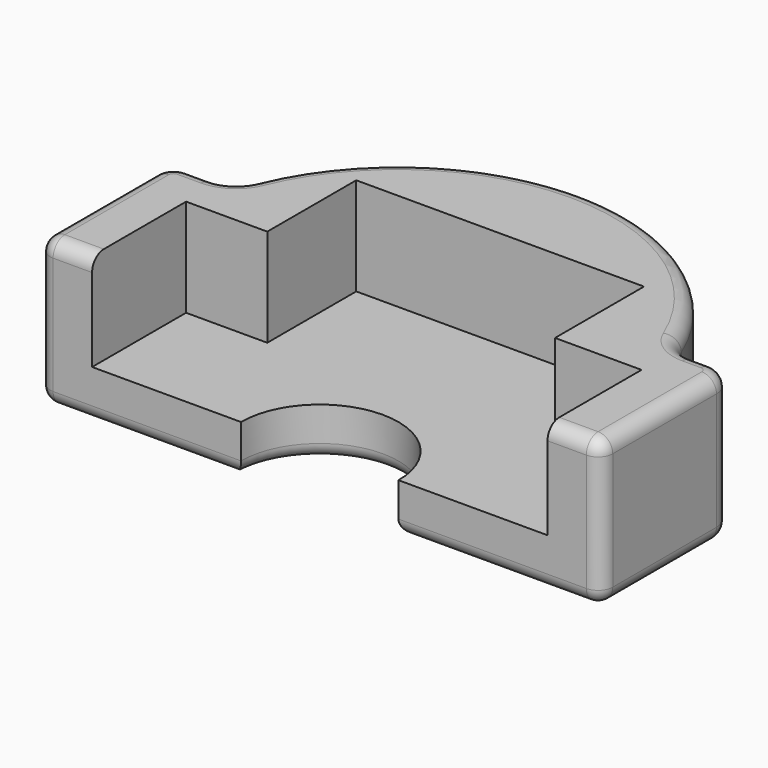
from build123d import *

# Parameters (mm, degrees)
F1_DEPTH     = 3.81
F2_R         = 0.762
F3_R         = 0.508
F4_R         = 0.381
F5_T1_DEPTH  = 0.6101247647
F5_T3_DEPTH  = 3.3655
F5_T5_DEPTH  = 5.8289214894
F5_T7_DEPTH  = 0.4831247647
F5_T9_DEPTH  = 5.8289214894
F5_T11_DEPTH = 3.048
F5_S15_W     = 0.381
F5_S15_H     = 0.381
F5_T16_DEPTH = 0.381
F5_S21_W     = 0.381
F5_S21_H     = 0.381
F5_T22_DEPTH = 0.381
F5_S27_W     = 0.381
F5_S27_H     = 0.381
F5_T28_DEPTH = 0.381
F5_S33_W     = 0.381
F5_S33_H     = 0.381
F5_T34_DEPTH = 0.381
F5_T38_ANGLE = 90
F5_T40_ANGLE = 67.60378922
F5_T42_ANGLE = 135.20757844
F5_T44_ANGLE = 67.60378922
F5_T46_ANGLE = 233.4571121673
F5_T48_ANGLE = 90
F7_DEPTH     = 2.54


# Not quite as in the source:
# - a fillet or chamfer that OpenCascade refuses, or shapes differently, is made with other operations: its cross-section is extruded or revolved along the edge and cut away or added


with BuildPart() as f1:
    # F0 (on Top) → F1 (new body)
    with BuildSketch(Plane.XY):
        with BuildLine():
            Line((0, -4.2545), (0, -8.509))
            Line((0, -8.509), (5.2574214894, -8.509))
            ThreePointArc((5.2574214894, -8.509), (7.3025, -6.4639214894), (9.3475785106, -8.509))
            Line((9.3475785106, -8.509), (14.605, -8.509))
            Line((14.605, -8.509), (14.605, -4.2545))
            Line((14.605, -4.2545), (13.081, -4.2545))
            ThreePointArc((13.081, -4.2545), (7.366, -0.0716128896), (1.651, -4.2545))
            Line((1.651, -4.2545), (0, -4.2545))
        make_face()
    extrude(amount=F1_DEPTH)

    # F2
    f2_edges = [f1.edges().sort_by_distance(p)[0] for p in [
        (13.081, -4.2545, 1.905),
        (1.651, -4.2545, 1.905),
    ]]
    fillet(f2_edges, radius=F2_R)

    # F3
    f3_edges = [f1.edges().sort_by_distance(p)[0] for p in [
        (0, -4.2545, 1.905),
        (14.605, -4.2545, 1.905),
    ]]
    fillet(f3_edges, radius=F3_R)

    # F4
    f4_edges = [f1.edges().sort_by_distance(p)[0] for p in [
        (0.813062, -4.2545, 0),
        (0.14879, -4.40329, 0),
        (1.542043, -4.125696, 0),
        (0, -6.63575, 0),
        (7.366, -0.071613, 0),
        (2.628711, -8.509, 0),
        (13.189957, -4.125696, 0),
        (7.3025, -6.463921, 0),
        (13.855438, -4.2545, 0),
        (11.976289, -8.509, 0),
        (14.45621, -4.40329, 0),
        (14.605, -6.63575, 0),
    ]]
    fillet(f4_edges, radius=F4_R)

    # F5: fillet of radius 0.381 on 14 edges, made by hand

    # F5_s2 → F5_t1 (cut)
    with BuildSketch(Plane.YZ.offset(0.508)):
        with BuildLine():
            ThreePointArc((-4.2545, 3.429), (-4.3660923164, 3.6984076836), (-4.6355, 3.81))
            Line((-4.6355, 3.81), (-4.2545, 3.81))
            Line((-4.2545, 3.81), (-4.2545, 3.429))
        make_face()
    extrude(amount=F5_T1_DEPTH, mode=Mode.SUBTRACT)

    # F5_s4 → F5_t3 (cut)
    with BuildSketch(Plane.XZ.offset(4.7625)):
        with BuildLine():
            ThreePointArc((0.381, 3.81), (0.1115923164, 3.6984076836), (0, 3.429))
            Line((0, 3.429), (0, 3.81))
            Line((0, 3.81), (0.381, 3.81))
        make_face()
        with BuildLine():
            ThreePointArc((14.224, 3.81), (14.4934076836, 3.6984076836), (14.605, 3.429))
            Line((14.605, 3.429), (14.605, 3.81))
            Line((14.605, 3.81), (14.224, 3.81))
        make_face()
    extrude(amount=F5_T3_DEPTH, mode=Mode.SUBTRACT)

    # F5_s6 → F5_t5 (cut)
    with BuildSketch(Plane.YZ.offset(0.381)):
        with BuildLine():
            ThreePointArc((-8.128, 3.81), (-8.3974076836, 3.6984076836), (-8.509, 3.429))
            Line((-8.509, 3.429), (-8.509, 3.81))
            Line((-8.509, 3.81), (-8.128, 3.81))
        make_face()
    extrude(amount=F5_T5_DEPTH, mode=Mode.SUBTRACT)

    # F5_s8 → F5_t7 (cut)
    with BuildSketch(Plane.YZ.offset(13.6138752353)):
        with BuildLine():
            ThreePointArc((-4.6355, 3.81), (-4.3660923164, 3.6984076836), (-4.2545, 3.429))
            Line((-4.2545, 3.429), (-4.2545, 3.81))
            Line((-4.2545, 3.81), (-4.6355, 3.81))
        make_face()
    extrude(amount=F5_T7_DEPTH, mode=Mode.SUBTRACT)

    # F5_s10 → F5_t9 (cut)
    with BuildSketch(Plane.YZ.offset(8.3950785106)):
        with BuildLine():
            ThreePointArc((-8.128, 3.81), (-8.3974076836, 3.6984076836), (-8.509, 3.429))
            Line((-8.509, 3.429), (-8.509, 3.81))
            Line((-8.509, 3.81), (-8.128, 3.81))
        make_face()
    extrude(amount=F5_T9_DEPTH, mode=Mode.SUBTRACT)

    # F5_s12 → F5_t11 (cut)
    with BuildSketch(Plane.XY.offset(0.381)):
        with BuildLine():
            ThreePointArc((0, -8.128), (0.1115923164, -8.3974076836), (0.381, -8.509))
            Line((0.381, -8.509), (0, -8.509))
            Line((0, -8.509), (0, -8.128))
        make_face()
        with BuildLine():
            ThreePointArc((14.224, -8.509), (14.4934076836, -8.3974076836), (14.605, -8.128))
            Line((14.605, -8.128), (14.605, -8.509))
            Line((14.605, -8.509), (14.224, -8.509))
        make_face()
    extrude(amount=F5_T11_DEPTH, mode=Mode.SUBTRACT)


with BuildPart() as f5_tool14:
    # F5_s15 → F5_t16 (new body)
    with BuildSketch(Plane.XZ.offset(8.128)):
        with Locations((14.4145, 0.1905)):
            Rectangle(F5_S15_W, F5_S15_H)
    extrude(amount=F5_T16_DEPTH)

    # F5_s17 → F5_t18 (revolve, cut)
    with BuildSketch(Plane(origin=(14.224, -8.128, 0.381), x_dir=(-0.7071067812, 0, 0.7071067812), z_dir=(0.7071067812, 0, 0.7071067812))):
        with BuildLine():
            ThreePointArc((0, -0.381), (0.381, 0), (0, 0.381))
            Line((0, 0.381), (0, -0.381))
        make_face()
    revolve(axis=Axis((14.224, -8.128, 0.381), (0, -1, 0)), mode=Mode.SUBTRACT)


with BuildPart() as f1_1:
    add(f1.part)

    # F5_t13: cut F5_tool14
    add(f5_tool14.part, mode=Mode.SUBTRACT)


with BuildPart() as f5_tool20:
    # F5_s21 → F5_t22 (new body)
    with BuildSketch(Plane.YZ.offset(0.381)):
        with Locations((-8.3185, 0.1905)):
            Rectangle(F5_S21_W, F5_S21_H)
    extrude(amount=-F5_T22_DEPTH)

    # F5_s23 → F5_t24 (revolve, cut)
    with BuildSketch(Plane(origin=(0.381, -8.128, 0.381), x_dir=(0, 0.7071067812, 0.7071067812), z_dir=(0, -0.7071067812, 0.7071067812))):
        with BuildLine():
            ThreePointArc((0, -0.381), (0.381, 0), (0, 0.381))
            Line((0, 0.381), (0, -0.381))
        make_face()
    revolve(axis=Axis((0.381, -8.128, 0.381), (-1, 0, 0)), mode=Mode.SUBTRACT)


with BuildPart() as f1_2:
    add(f1_1.part)

    # F5_t19: cut F5_tool20
    add(f5_tool20.part, mode=Mode.SUBTRACT)


with BuildPart() as f5_tool26:
    # F5_s27 → F5_t28 (new body)
    with BuildSketch(Plane.XZ.offset(8.128)):
        with Locations((0.1905, 3.6195)):
            Rectangle(F5_S27_W, F5_S27_H)
    extrude(amount=F5_T28_DEPTH)

    # F5_s29 → F5_t30 (revolve, cut)
    with BuildSketch(Plane(origin=(0.381, -8.128, 3.429), x_dir=(0.7071067812, 0, -0.7071067812), z_dir=(-0.7071067812, 0, -0.7071067812))):
        with BuildLine():
            ThreePointArc((0, -0.381), (0.381, 0), (0, 0.381))
            Line((0, 0.381), (0, -0.381))
        make_face()
    revolve(axis=Axis((0.381, -8.128, 3.429), (0, -1, 0)), mode=Mode.SUBTRACT)


with BuildPart() as f1_3:
    add(f1_2.part)

    # F5_t25: cut F5_tool26
    add(f5_tool26.part, mode=Mode.SUBTRACT)


with BuildPart() as f5_tool32:
    # F5_s33 → F5_t34 (new body)
    with BuildSketch(Plane.YZ.offset(14.224)):
        with Locations((-8.3185, 3.6195)):
            Rectangle(F5_S33_W, F5_S33_H)
    extrude(amount=F5_T34_DEPTH)

    # F5_s35 → F5_t36 (revolve, cut)
    with BuildSketch(Plane(origin=(14.224, -8.128, 3.429), x_dir=(0, 0.7071067812, -0.7071067812), z_dir=(0, -0.7071067812, -0.7071067812))):
        with BuildLine():
            ThreePointArc((0, -0.381), (0.381, 0), (0, 0.381))
            Line((0, 0.381), (0, -0.381))
        make_face()
    revolve(axis=Axis((14.224, -8.128, 3.429), (1, 0, 0)), mode=Mode.SUBTRACT)


with BuildPart() as f1_4:
    add(f1_3.part)

    # F5_t31: cut F5_tool32
    add(f5_tool32.part, mode=Mode.SUBTRACT)

    # F5_s37 → F5_t38 (revolve, cut)
    with BuildSketch(Plane.YZ.offset(0.508)):
        with BuildLine():
            ThreePointArc((-4.2545, 3.429), (-4.3660923164, 3.6984076836), (-4.6355, 3.81))
            Line((-4.6355, 3.81), (-4.2545, 3.81))
            Line((-4.2545, 3.81), (-4.2545, 3.429))
        make_face()
    revolve(axis=Axis((0.508, -4.7625, 3.81), (0, 0, 1)), revolution_arc=F5_T38_ANGLE, mode=Mode.SUBTRACT)

    # F5_s39 → F5_t40 (revolve, cut)
    with BuildSketch(Plane.YZ.offset(1.1181247647)):
        with BuildLine():
            ThreePointArc((-4.6355, 3.81), (-4.3660923164, 3.6984076836), (-4.2545, 3.429))
            Line((-4.2545, 3.429), (-4.2545, 3.81))
            Line((-4.2545, 3.81), (-4.6355, 3.81))
        make_face()
    revolve(axis=Axis((1.1181247647, -3.4925, 3.81), (0, 0, 1)), revolution_arc=F5_T40_ANGLE, mode=Mode.SUBTRACT)

    # F5_s41 → F5_t42 (revolve, cut)
    with BuildSketch(Plane(origin=(3.2066030929, -7.7812628503, 0), x_dir=(0, 0, 1), z_dir=(0.3810092313, -0.9245712334, 0))):
        with BuildLine():
            ThreePointArc((3.81, -10.113322678), (3.6984076836, -10.3827303617), (3.429, -10.494322678))
            Line((3.429, -10.494322678), (3.81, -10.494322678))
            Line((3.81, -10.494322678), (3.81, -10.113322678))
        make_face()
    revolve(axis=Axis((7.366, -6.0672049597, 3.81), (0, 0, 1)), revolution_arc=F5_T42_ANGLE, mode=Mode.SUBTRACT)

    # F5_s43 → F5_t44 (revolve, cut)
    with BuildSketch(Plane.YZ.offset(13.6138752353)):
        with BuildLine():
            ThreePointArc((-4.6355, 3.81), (-4.3660923164, 3.6984076836), (-4.2545, 3.429))
            Line((-4.2545, 3.429), (-4.2545, 3.81))
            Line((-4.2545, 3.81), (-4.6355, 3.81))
        make_face()
    revolve(axis=Axis((13.6138752353, -3.4925, 3.81), (0, 0, -1)), revolution_arc=F5_T44_ANGLE, mode=Mode.SUBTRACT)

    # F5_s45 → F5_t46 (revolve, cut)
    with BuildSketch(Plane(origin=(4.8953206605, -9.721188669, 0), x_dir=(0, 0, 1), z_dir=(0.449764197, -0.8931473378, 0))):
        with BuildLine():
            ThreePointArc((3.81, -0.2690863714), (3.6984076836, -0.5384940551), (3.429, -0.6500863714))
            Line((3.429, -0.6500863714), (3.81, -0.6500863714))
            Line((3.81, -0.6500863714), (3.81, -0.2690863714))
        make_face()
    revolve(axis=Axis((7.3025, -8.509, 3.81), (0, 0, -1)), revolution_arc=F5_T46_ANGLE, mode=Mode.SUBTRACT)

    # F5_s47 → F5_t48 (revolve, cut)
    with BuildSketch(Plane.YZ.offset(14.097)):
        with BuildLine():
            ThreePointArc((-4.6355, 3.81), (-4.3660923164, 3.6984076836), (-4.2545, 3.429))
            Line((-4.2545, 3.429), (-4.2545, 3.81))
            Line((-4.2545, 3.81), (-4.6355, 3.81))
        make_face()
    revolve(axis=Axis((14.097, -4.7625, 3.81), (0, 0, -1)), revolution_arc=F5_T48_ANGLE, mode=Mode.SUBTRACT)

    # F6 (on face) → F7 (cut)
    with BuildSketch(Plane.XY.offset(3.81)):
        Polygon((1.3930101413, -5.4594320245), (1.3930101413, -8.8049108163), (1.3930101413, -9.2631950974), (13.2167544216, -9.2631950974), (13.2167544216, -5.4594320245), (10.9711596742, -5.4594320245), (10.9711596742, -2.5722389109), (3.5011197906, -2.5722389109), (3.5011197906, -5.4594320245), align=None)
    extrude(amount=-F7_DEPTH, mode=Mode.SUBTRACT)


solid = f1_4.part
